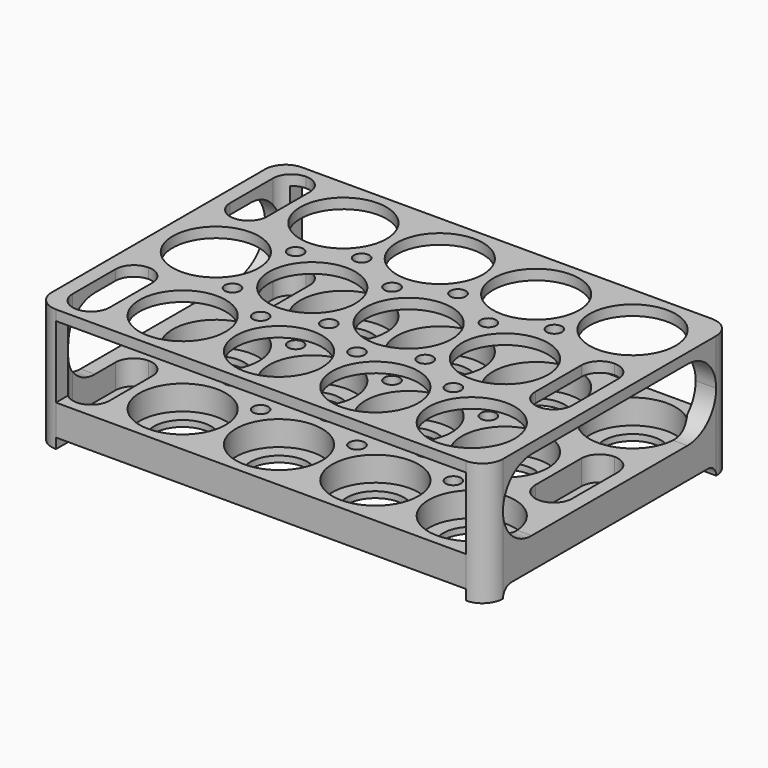
from build123d import *

# Parameters (mm, degrees)
F1_DEPTH = 139.7
F2_W     = 127
F2_H     = 22.225
F2_H_2   = 3.175
F3_DEPTH = 95.251
F4_R     = 13.335
F4_R_2   = 2.38125
F5_DEPTH = 33.02
F6_R     = 6.34999
F7_R     = 8.89
F8_DEPTH = 12.7
F9_R     = 3.17499


# Not quite as in the source:
# - a fillet or chamfer is up to 0.001 mm smaller than in the source, because OpenCascade refuses the exact size
# - a feature names something its author has since deleted; it is built from what else it names


with BuildPart() as f1:
    # F0 (on Right) → F1 (new body)
    with BuildSketch(Plane.YZ):
        Polygon((41.275, -19.05), (47.625, -19.05), (47.625, 19.05), (-47.625, 19.05), (-47.625, -19.05), (-41.275, -19.05), (-41.275, -15.875), (41.275, -15.875), align=None)
        with BuildLine():
            Line((30.1625, -6.35), (-30.1625, -6.35))
            ThreePointArc((-30.1625, -6.35), (-38.0202241059, -3.0952241059), (-41.275, 4.7625))
            ThreePointArc((-41.275, 4.7625), (-38.0202241059, 12.6202241059), (-30.1625, 15.875))
            Line((-30.1625, 15.875), (30.1625, 15.875))
            ThreePointArc((30.1625, 15.875), (38.0202241059, 12.6202241059), (41.275, 4.7625))
            ThreePointArc((41.275, 4.7625), (38.0202241059, -3.0952241059), (30.1625, -6.35))
        make_face(mode=Mode.SUBTRACT)
    extrude(amount=F1_DEPTH)

    # F2 (on face) → F3 (cut, through all)
    with BuildSketch(Plane(origin=(0, 47.625, 0), x_dir=(-1, 0, 0), z_dir=(0, 1, 0))):
        with Locations((-69.85, 4.7625)):
            Rectangle(F2_W, F2_H)
        with Locations((-69.85, -17.4625)):
            Rectangle(F2_W, F2_H_2)
    extrude(amount=-F3_DEPTH, mode=Mode.SUBTRACT)

    # F4 (on face) → F5 (cut)
    with BuildSketch(Plane.XY.offset(19.05)):
        with Locations((121.92, -31.115)):
            Circle(F4_R)
        with Locations((92.075, -31.115)):
            Circle(F4_R)
        with Locations((62.23, -31.115)):
            Circle(F4_R)
        with Locations((32.385, -31.115)):
            Circle(F4_R)
        with Locations((17.78, 0)):
            Circle(F4_R)
        with Locations((47.625, 0)):
            Circle(F4_R)
        with Locations((77.47, 0)):
            Circle(F4_R)
        with Locations((107.315, 0)):
            Circle(F4_R)
        with Locations((121.92, 31.115)):
            Circle(F4_R)
        with Locations((92.075, 31.115)):
            Circle(F4_R)
        with Locations((62.23, 31.115)):
            Circle(F4_R)
        with Locations((32.385, 31.115)):
            Circle(F4_R)
        with BuildLine():
            ThreePointArc((10.16, 16.51), (14.2011152545, 18.1838847455), (15.875, 22.225))
            Line((15.875, 22.225), (15.875, 38.735))
            ThreePointArc((15.875, 38.735), (14.2011152545, 42.7761152545), (10.16, 44.45))
            ThreePointArc((10.16, 44.45), (6.1188847455, 42.7761152545), (4.445, 38.735))
            Line((4.445, 38.735), (4.445, 22.225))
            ThreePointArc((4.445, 22.225), (6.1188847455, 18.1838847455), (10.16, 16.51))
        make_face()
        with Locations((106.9762696236, 19.558)):
            Circle(F4_R_2)
        with Locations((92.4001972518, 12.2265492083)):
            Circle(F4_R_2)
        with Locations((77.1312696236, 19.558)):
            Circle(F4_R_2)
        with Locations((62.5551972518, 12.2265492083)):
            Circle(F4_R_2)
        with Locations((47.2862696236, 19.558)):
            Circle(F4_R_2)
        with Locations((32.7101972518, 12.2265492083)):
            Circle(F4_R_2)
        with Locations((32.7101972518, -12.2265492083)):
            Circle(F4_R_2)
        with Locations((47.2862696236, -19.558)):
            Circle(F4_R_2)
        with Locations((62.5551972518, -12.2265492083)):
            Circle(F4_R_2)
        with Locations((77.1312696236, -19.558)):
            Circle(F4_R_2)
        with Locations((92.4001972518, -12.2265492083)):
            Circle(F4_R_2)
        with Locations((106.9762696236, -19.558)):
            Circle(F4_R_2)
        with BuildLine():
            ThreePointArc((10.16, -44.45), (14.2011152545, -42.7761152545), (15.875, -38.735))
            Line((15.875, -38.735), (15.875, -22.225))
            ThreePointArc((15.875, -22.225), (14.2011152545, -18.1838847455), (10.16, -16.51))
            ThreePointArc((10.16, -16.51), (6.1188847455, -18.1838847455), (4.445, -22.225))
            Line((4.445, -22.225), (4.445, -38.735))
            ThreePointArc((4.445, -38.735), (6.1188847455, -42.7761152545), (10.16, -44.45))
        make_face()
        with BuildLine():
            ThreePointArc((129.54, -14.605), (133.5811152545, -12.9311152545), (135.255, -8.89))
            Line((135.255, -8.89), (135.255, 8.89))
            ThreePointArc((135.255, 8.89), (133.5811152545, 12.9311152545), (129.54, 14.605))
            ThreePointArc((129.54, 14.605), (125.4988847455, 12.9311152545), (123.825, 8.89))
            Line((123.825, 8.89), (123.825, -8.89))
            ThreePointArc((123.825, -8.89), (125.4988847455, -12.9311152545), (129.54, -14.605))
        make_face()
    extrude(amount=-F5_DEPTH, mode=Mode.SUBTRACT)

    # F6 (radius 6.35 in the source; OpenCascade refuses exactly that, so slightly less here)
    f6_edges = [f1.edges().sort_by_distance(p)[0] for p in [
        (0, 47.625, 0),
        (0, -47.625, 0),
        (139.7, -47.625, 0),
        (139.7, 47.625, 0),
    ]]
    fillet(f6_edges, radius=F6_R)

    # F7 (on face) → F8 (cut, symmetric)
    with BuildSketch(Plane(origin=(0, 0, -15.875), x_dir=(1, 0, 0), z_dir=(0, 0, -1))):
        with Locations((17.78, 0)):
            Circle(F7_R)
        with Locations((47.625, 0)):
            Circle(F7_R)
        with Locations((77.47, 0)):
            Circle(F7_R)
        with Locations((107.315, 0)):
            Circle(F7_R)
        with Locations((121.92, -31.115)):
            Circle(F7_R)
        with Locations((92.075, -31.115)):
            Circle(F7_R)
        with Locations((62.23, -31.115)):
            Circle(F7_R)
        with Locations((32.385, -31.115)):
            Circle(F7_R)
        with Locations((32.385, 31.115)):
            Circle(F7_R)
        with Locations((62.23, 31.115)):
            Circle(F7_R)
        with Locations((92.075, 31.115)):
            Circle(F7_R)
        with Locations((121.92, 31.115)):
            Circle(F7_R)
    extrude(amount=F8_DEPTH, both=True, mode=Mode.SUBTRACT)

    # F9 (radius 3.175 in the source; OpenCascade refuses exactly that, so slightly less here)
    f9_edges = [f1.edges().sort_by_distance(p)[0] for p in [
        (136.525, -41.275, -15.875),
        (136.525, 41.275, -15.875),
        (3.175, 41.275, -15.875),
        (3.175, -41.275, -15.875),
    ]]
    fillet(f9_edges, radius=F9_R)


solid = f1.part
